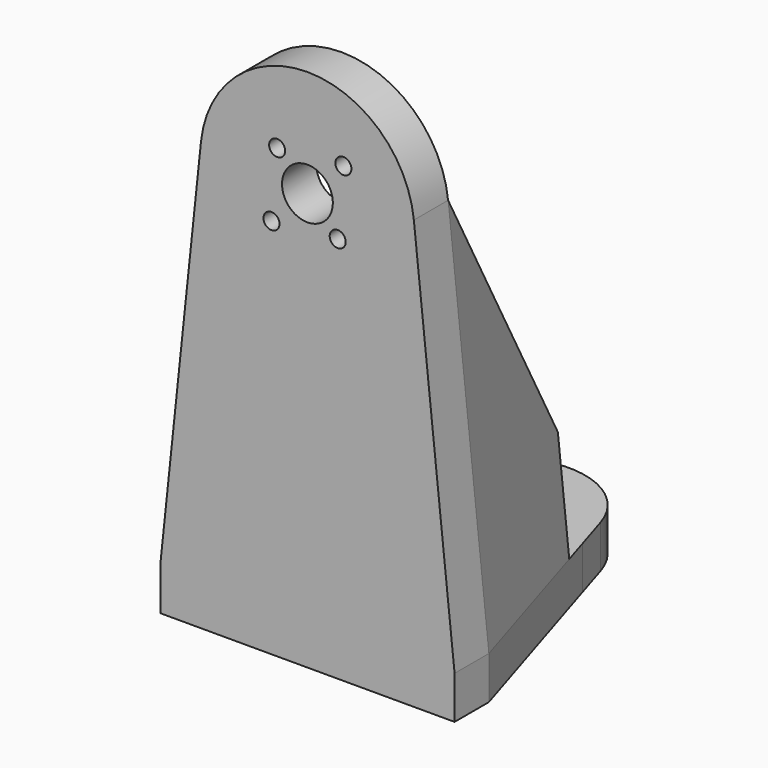
from build123d import *

# Parameters (mm, degrees)
F0_R      = 1.5
F0_R_2    = 2.5
F1_DEPTH  = 8
F2_W      = 55
F2_H      = 8
F3_DEPTH  = 8
F4_R      = 4.75
F4_R_2    = 1.5
F5_DEPTH  = 8
F8_REACH  = 140.1940387091
F11_REACH = 140.1940387091
F13_DEPTH = 25


with BuildPart() as f1:
    # F0 (on Top) → F1 (new body)
    with BuildSketch(Plane.XY):
        Polygon((-27.5, 8), (-27.5, 0), (27.5, 0), (27.5, 8), (19.1259515677, 8), (-19.1259515677, 8), align=None)
        with BuildLine():
            Line((-16.4747191004, 43.64), (-27.5, 8))
            Line((-27.5, 8), (-19.1259515677, 8))
            Line((-19.1259515677, 8), (-9.6474272477, 38.64))
            Line((-9.6474272477, 38.64), (9.6474272477, 38.64))
            Line((9.6474272477, 38.64), (19.1259515677, 8))
            Line((19.1259515677, 8), (27.5, 8))
            Line((27.5, 8), (16.4747191004, 43.64))
            Line((16.4747191004, 43.64), (14.3299863823, 50.5730001446))
            ThreePointArc((14.3299863823, 50.5730001446), (0, 61.14), (-14.3299863823, 50.5730001446))
            Line((-14.3299863823, 50.5730001446), (-16.4747191004, 43.64))
        make_face()
        with Locations((-10, 46.14)):
            Circle(F0_R, mode=Mode.SUBTRACT)
        with Locations((0, 46.14)):
            Circle(F0_R_2, mode=Mode.SUBTRACT)
        with Locations((10, 46.14)):
            Circle(F0_R, mode=Mode.SUBTRACT)
    extrude(amount=F1_DEPTH)

    # F2 (on face) → F3 (join)
    with BuildSketch(Plane.XZ):
        with BuildLine():
            Line((27.5, 8), (19.8895027624, 80.0994475138))
            ThreePointArc((19.8895027624, 80.0994475138), (0, 98), (-19.8895027624, 80.0994475138))
            Line((-19.8895027624, 80.0994475138), (-27.5, 8))
            Line((-27.5, 8), (27.5, 8))
        make_face()
        with Locations((0, 4)):
            Rectangle(F2_W, F2_H)
    extrude(amount=-F3_DEPTH)

    # F4 (on face) → F5 (cut, through all)
    with BuildSketch(Plane.XZ):
        with Locations((0, 78)):
            Circle(F4_R)
        with Locations((-5.6568542495, 83.6568542495)):
            Circle(F4_R_2)
        with Locations((6.7175144213, 84.7175144213)):
            Circle(F4_R_2)
        with Locations((5.6568542495, 72.3431457505)):
            Circle(F4_R_2)
        with Locations((-6.7175144213, 71.2824855787)):
            Circle(F4_R_2)
    extrude(amount=-F5_DEPTH, mode=Mode.SUBTRACT)

    f8_end = Plane(origin=(14.3866894077, 23.32, 4), x_dir=(0.295533343, -0.9553324255, 0), z_dir=(-0.9553324255, -0.295533343, 0))
    # F7 (on 3pt) → F8 (join, up to a plane its end follows)
    with BuildSketch(Plane(origin=(27.8443578743, 8.6136887495, 2.9391266645), x_dir=(-0.2924175497, 0.9557924714, -0.0308662969), z_dir=(0.95051185, 0.2940420916, 0.1003318064))):
        Polygon((-0.6420732198, 77.5690607735), (-0.6420732198, 5.0690607735), (43.900022914, 6.4515483908), align=None)
    f8_long = extrude(amount=-F8_REACH, mode=Mode.PRIVATE)
    add(split(f8_long, bisect_by=f8_end, keep=Keep.BOTTOM, mode=Mode.PRIVATE))

    f11_end = Plane(origin=(-14.3866894077, 23.32, 4), x_dir=(0.295533343, 0.9553324255, 0), z_dir=(0.9553324255, -0.295533343, 0))
    # F10 (on 3pt) → F11 (join, up to a plane its end follows)
    with BuildSketch(Plane(origin=(-27.8443578743, 8.6136887495, 2.9391266645), x_dir=(0.2924175497, 0.9557924714, -0.0308662969), z_dir=(0.95051185, -0.2940420916, -0.1003318064))):
        Polygon((-0.6420732198, 77.5690607735), (-0.6420732198, 5.0690607735), (43.900022914, 6.4515483908), align=None)
    f11_long = extrude(amount=F11_REACH, mode=Mode.PRIVATE)
    add(split(f11_long, bisect_by=f11_end, keep=Keep.BOTTOM, mode=Mode.PRIVATE))

    # F12 (on face) → F13 (cut)
    with BuildSketch(Plane.XY.offset(8)):
        with BuildLine():
            Line((-18.02147568, 38.64), (-9.6474272477, 38.64))
            Line((-9.6474272477, 38.64), (9.6474272477, 38.64))
            Line((9.6474272477, 38.64), (18.02147568, 38.64))
            Line((18.02147568, 38.64), (14.3299863823, 50.5730001446))
            ThreePointArc((14.3299863823, 50.5730001446), (0, 61.14), (-14.3299863823, 50.5730001446))
            Line((-14.3299863823, 50.5730001446), (-18.02147568, 38.64))
        make_face()
    extrude(amount=F13_DEPTH, mode=Mode.SUBTRACT)


solid = f1.part
